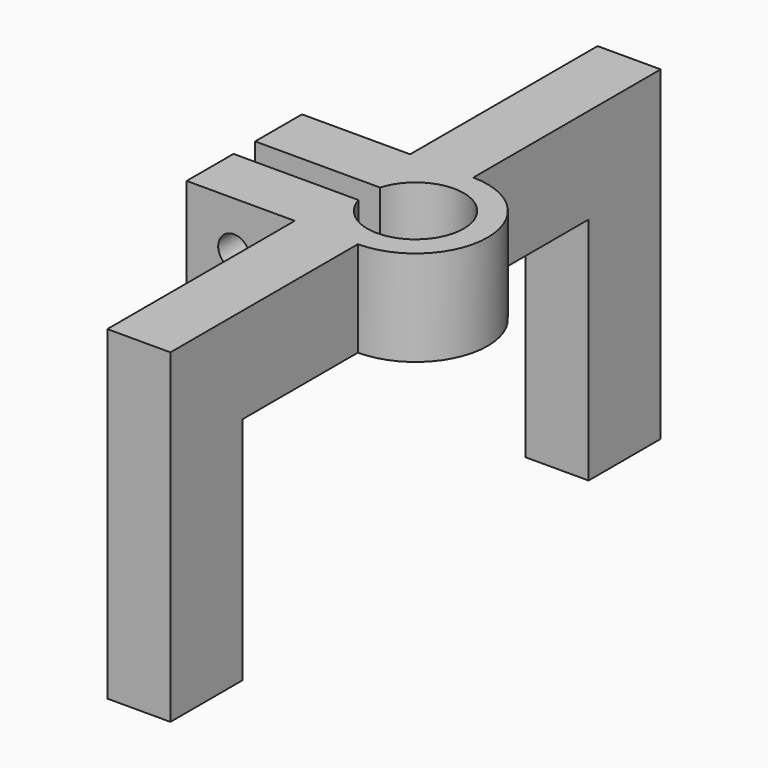
from build123d import *

# Parameters (mm, degrees)
F0_R      = 8
F1_DEPTH  = 10.6
F2_W      = 19
F2_H      = 6.5
F3_DEPTH  = 10.6
F4_R      = 5.35
F5_DEPTH  = 10.601
F6_W      = 5.4454011573
F6_H      = 3
F7_DEPTH  = 10.601
F8_R      = 1.75
F9_DEPTH  = 16.001
F10_W     = 7
F10_H     = 10.6
F11_DEPTH = 26
F12_W     = 7
F12_H     = 10
F13_DEPTH = 25.5
F14_W     = 7
F14_H     = 10.6
F15_DEPTH = 26
F16_W     = 7
F16_H     = 10
F17_DEPTH = 25.5
F18_R     = 1.75
F19_DEPTH = 10


with BuildPart() as f1:
    # F0 (on Top) → F1 (new body)
    with BuildSketch(Plane.XY):
        Circle(F0_R)
    extrude(amount=-F1_DEPTH)

    # F2 (on face) → F3 (join, through all)
    with BuildSketch(Plane.XY):
        with Locations((-9.5, 4.75)):
            Rectangle(F2_W, F2_H)
        with Locations((-9.5, -4.75)):
            Rectangle(F2_W, F2_H)
    extrude(amount=-F3_DEPTH)

    # F4 (on face) → F5 (cut, through all)
    with BuildSketch(Plane.XY):
        Circle(F4_R)
    extrude(amount=-F5_DEPTH, mode=Mode.SUBTRACT)

    # F6 (on face) → F7 (cut, through all)
    with BuildSketch(Plane.XY):
        with Locations((-7.8581168228, 0)):
            Rectangle(F6_W, F6_H)
    extrude(amount=-F7_DEPTH, mode=Mode.SUBTRACT)

    # F8 (on face) → F9 (cut, through all)
    with BuildSketch(Plane.XZ.offset(8)):
        with Locations((-13.75, -5.25)):
            Circle(F8_R)
    extrude(amount=-F9_DEPTH, mode=Mode.SUBTRACT)

    # F10 (on face) → F11 (join)
    with BuildSketch(Plane.XZ.offset(8)):
        with Locations((-3.5, -5.3)):
            Rectangle(F10_W, F10_H)
    extrude(amount=F11_DEPTH)

    # F12 (on face) → F13 (join)
    with BuildSketch(Plane(origin=(0, 0, -10.6), x_dir=(1, 0, 0), z_dir=(0, 0, -1))):
        with Locations((-3.5, 29)):
            Rectangle(F12_W, F12_H)
    extrude(amount=F13_DEPTH)

    # F14 (on face) → F15 (join)
    with BuildSketch(Plane(origin=(0, 8, 0), x_dir=(-1, 0, 0), z_dir=(0, 1, 0))):
        with Locations((3.5, -5.3)):
            Rectangle(F14_W, F14_H)
    extrude(amount=F15_DEPTH)

    # F16 (on face) → F17 (join)
    with BuildSketch(Plane(origin=(0, 0, -10.6), x_dir=(1, 0, 0), z_dir=(0, 0, -1))):
        with Locations((-3.5, -29)):
            Rectangle(F16_W, F16_H)
    extrude(amount=F17_DEPTH)

    # F18 (on face) → F19 (cut)
    with BuildSketch(Plane(origin=(0, 0, -36.1), x_dir=(1, 0, 0), z_dir=(0, 0, -1))):
        with Locations((-3.5, 29)):
            Circle(F18_R)
        with Locations((-3.5, -29)):
            Circle(F18_R)
    extrude(amount=-F19_DEPTH, mode=Mode.SUBTRACT)


solid = f1.part
